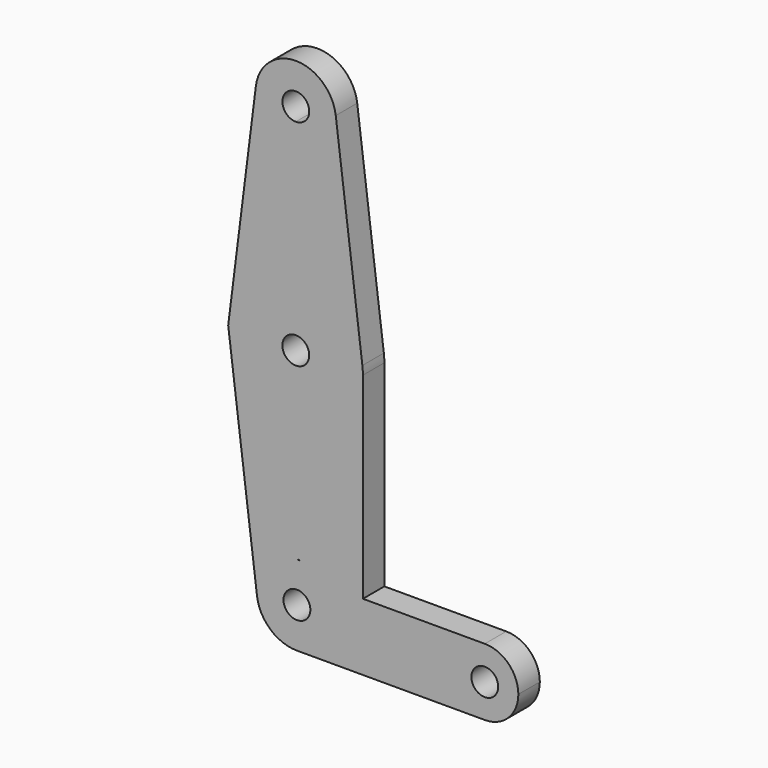
from build123d import *

# Parameters (mm, degrees)
F0_R     = 3.175
F1_DEPTH = 6.35


# Not quite as in the source:
# - the program builds the solid bodies; features that only make, move or delete a surface that nothing else refers to are left out


with BuildPart() as f1:
    # F0 (on Front) → F1 (new body)
    with BuildSketch(Plane.XZ):
        with BuildLine():
            ThreePointArc((15.7504882737, 1.984375), (10.5003255158, 11.90625), (0, 15.875))
            ThreePointArc((0, 15.875), (-10.500325544, 11.9062499751), (-15.7504882831, 1.9843749253))
            ThreePointArc((-15.7504882831, 1.9843749253), (-15.875, -5.44e-08), (-15.7504882695, -1.9843750333))
            ThreePointArc((-15.7504882695, -1.9843750333), (0.9941387534, -15.8438414893), (15.875, 0))
            ThreePointArc((15.875, 0), (15.8440389276, 0.9909871135), (15.7512764776, 1.9781087752))
            ThreePointArc((15.7512764776, 1.9781087752), (15.7508826872, 1.9812419268), (15.7504882737, 1.984375))
        make_face()
        with BuildLine():
            ThreePointArc((0, 3.175), (2.2450640303, 2.2450640303), (3.175, 0))
            ThreePointArc((3.175, 0), (-2.2450640303, -2.2450640303), (0, 3.175))
        make_face(mode=Mode.SUBTRACT)
        with BuildLine():
            ThreePointArc((-15.7504882831, 1.9843749253), (-10.500325544, 11.9062499751), (0, 15.875))
            Line((0, 15.875), (0, 41.275))
            ThreePointArc((0, 41.275), (-7.14375, 44.4998046905), (-9.4502929642, 51.990625))
            Line((-9.4502929642, 51.990625), (-15.7504882831, 1.9843749253))
        make_face()
        with BuildLine():
            Line((0, 41.275), (0, 15.875))
            ThreePointArc((0, 15.875), (10.5003255158, 11.90625), (15.7504882737, 1.984375))
            Line((15.7504882737, 1.984375), (9.4502929642, 51.990625))
            ThreePointArc((9.4502929642, 51.990625), (9.5063048942, 51.396483242), (9.525, 50.8))
            ThreePointArc((9.525, 50.8), (6.7351920908, 44.0648079092), (0, 41.275))
        make_face()
        with BuildLine():
            ThreePointArc((-15.7504882695, -1.9843750333), (-15.875, -5.44e-08), (-15.7504882831, 1.9843749253))
            Line((-15.7504882831, 1.9843749253), (-16.0004960241, 0))
            Line((-16.0004960241, 0), (-15.7504882695, -1.9843750333))
        make_face()
        with BuildLine():
            ThreePointArc((-9.4502929642, 51.990625), (-7.14375, 44.4998046905), (0, 41.275))
            ThreePointArc((0, 41.275), (6.7351920908, 44.0648079092), (9.525, 50.8))
            ThreePointArc((9.525, 50.8), (9.5063048942, 51.396483242), (9.4502929642, 51.990625))
            ThreePointArc((9.4502929642, 51.990625), (0, 60.325), (-9.4502929642, 51.990625))
        make_face()
        with BuildLine():
            ThreePointArc((3.175, 50.8), (2.2450640303, 48.5549359697), (0, 47.625))
            ThreePointArc((0, 47.625), (-2.2450640303, 53.0450640303), (3.175, 50.8))
        make_face(mode=Mode.SUBTRACT)
        with BuildLine():
            ThreePointArc((15.875, 0), (0.9941387534, -15.8438414893), (-15.7504882695, -1.9843750333))
            Line((-15.7504882695, -1.9843750333), (-9.182062028, -54.1196420534))
            ThreePointArc((-9.182062028, -54.1196420534), (-6.9635285808, -46.7300430021), (0, -43.4077945917))
            ThreePointArc((0, -43.4077945917), (0.9024529842, -43.4251553439), (1.7992106078, -43.5278614731))
            ThreePointArc((1.7992106078, -43.5278614731), (7.5245456473, -46.7588045924), (9.7932309362, -52.9290170534))
            ThreePointArc((9.7932309362, -52.9290170534), (7.003423027, -59.6642091442), (0.2682309362, -62.4540170534))
            Line((0.2682309362, -62.4540170534), (44.7182309362, -62.4540170534))
            ThreePointArc((44.7182309362, -62.4540170534), (36.7807309362, -54.5165170534), (44.7182309362, -46.5790170534))
            Line((44.7182309362, -46.5790170534), (15.875, -46.5790170534))
            Line((15.875, -46.5790170534), (15.875, 0))
        make_face()
        with BuildLine():
            ThreePointArc((0, -43.4077945917), (-6.9635285808, -46.7300430021), (-9.182062028, -54.1196420534))
            ThreePointArc((-9.182062028, -54.1196420534), (-6.0319643733, -60.0727670534), (0.2682309362, -62.4540170534))
            ThreePointArc((0.2682309362, -62.4540170534), (7.003423027, -59.6642091442), (9.7932309362, -52.9290170534))
            ThreePointArc((9.7932309362, -52.9290170534), (7.5245456473, -46.7588045924), (1.7992106078, -43.5278614731))
            Line((1.7992106078, -43.5278614731), (0, -43.4077945917))
        make_face()
        with Locations((0.2682309362, -52.9290170534)):
            Circle(F0_R, mode=Mode.SUBTRACT)
        with BuildLine():
            ThreePointArc((52.6557309362, -54.5165170534), (50.3308910119, -48.9038569777), (44.7182309362, -46.5790170534))
            ThreePointArc((44.7182309362, -46.5790170534), (36.7807309362, -54.5165170534), (44.7182309362, -62.4540170534))
            ThreePointArc((44.7182309362, -62.4540170534), (50.3308910119, -60.1291771291), (52.6557309362, -54.5165170534))
        make_face()
        with Locations((44.7182309362, -54.5165170534)):
            Circle(F0_R, mode=Mode.SUBTRACT)
    extrude(amount=F1_DEPTH)


solid = f1.part
